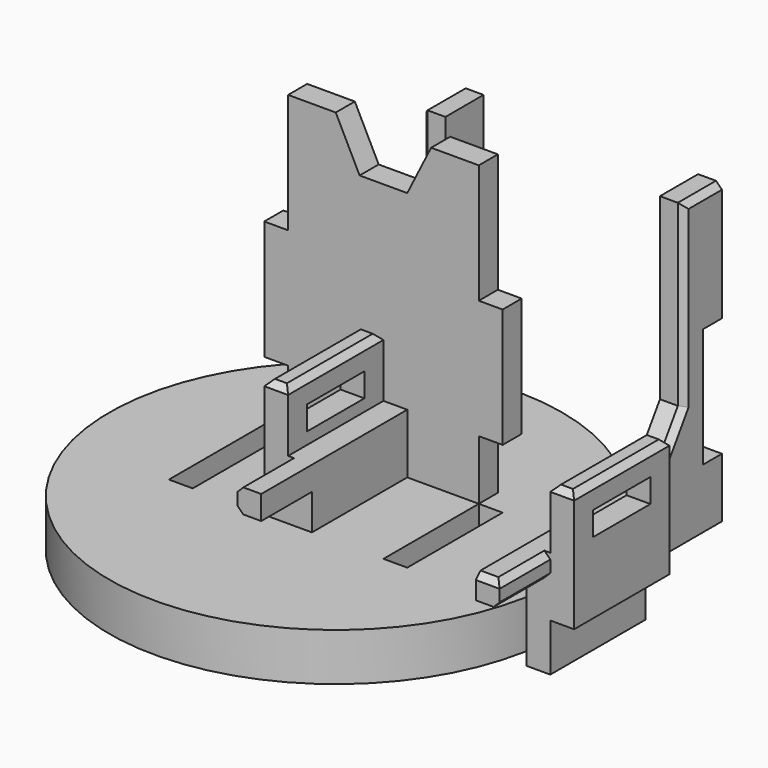
from build123d import *

# Parameters (mm, degrees)
F0_R       = 19
F1_DEPTH   = 4
F2_W       = 2
F2_H       = 10
F3_DEPTH   = 4.001
F5_DEPTH   = 2
F8_DEPTH   = 25
F9_W       = 2
F9_H       = 10
F9_H_2     = 5
F10_DEPTH  = 26.001
F6_W       = 2
F6_H       = 10
F11_DEPTH  = 19.001
F13_DEPTH  = 14.001
F15_W      = 10
F15_H      = 5
F16_DEPTH  = 2
F17_W      = 6
F17_H      = 2
F18_DEPTH  = 24.001
F19_W      = 10
F19_H      = 5
F20_DEPTH  = 2
F21_W      = 6
F21_H      = 2
F22_DEPTH  = 43.001
F23_SIZE   = 0.5
F23_2_SIZE = 0.5


with BuildPart() as f1:
    # F0 (on Top) → F1 (new body)
    with BuildSketch(Plane.XY):
        Circle(F0_R)
    extrude(amount=F1_DEPTH)

    # F2 (on face) → F3 (cut, through all)
    with BuildSketch(Plane.XY.offset(4)):
        with Locations((-9, 0)):
            Rectangle(F2_W, F2_H)
        with Locations((9, 0)):
            Rectangle(F2_W, F2_H)
    extrude(amount=-F3_DEPTH, mode=Mode.SUBTRACT)


with BuildPart() as f5:
    # F4 (on Right) → F5 (new body)
    with BuildSketch(Plane.YZ):
        Polygon((-5, 4), (-5, 0), (5, 0), (5, 4), (13, 4), (13, 29), (9, 29), (9, 14), (5.6833752096, 9), (-10.3166247904, 9), (-10.3166247904, 7), (-5, 7), align=None)
    extrude(amount=F5_DEPTH)

    # F6 (on face) → F11 (cut, through all)
    with BuildSketch(Plane(origin=(0, 0, 0), x_dir=(0, -1, 0), z_dir=(-1, 0, 0))):
        with Locations((-12, 14)):
            Rectangle(F6_W, F6_H)
    extrude(amount=-F11_DEPTH, mode=Mode.SUBTRACT)


with BuildPart() as f8:
    # F7 (on face) → F8 (new body)
    with BuildSketch(Plane.XY.offset(4)):
        Polygon((-10, 7), (-10, 5), (-8, 5), (8, 5), (10, 5), (10, 7), align=None)
    extrude(amount=F8_DEPTH)

    # F9 (on face) → F10 (cut, through all)
    with BuildSketch(Plane(origin=(0, 7, 0), x_dir=(-1, 0, 0), z_dir=(0, 1, 0))):
        with Locations((-9, 24)):
            Rectangle(F9_W, F9_H)
        with Locations((9, 24)):
            Rectangle(F9_W, F9_H)
        with Locations((9, 6.5)):
            Rectangle(F9_W, F9_H_2)
        with Locations((-9, 6.5)):
            Rectangle(F9_W, F9_H_2)
    extrude(amount=-F10_DEPTH, mode=Mode.SUBTRACT)

    # F12 (on face) → F13 (cut, through all)
    with BuildSketch(Plane.XZ.offset(-5)):
        Polygon((4, 29), (-4, 29), (-2, 25), (2, 25), align=None)
    extrude(amount=-F13_DEPTH, mode=Mode.SUBTRACT)


with BuildPart() as f14_1:
    # F14: copy of F5
    add(f5.part.moved(Location((20, 0, 0))))

    # F19 (on face) → F20 (join)
    with BuildSketch(Plane.YZ.offset(22)):
        with Locations((0, 11.5)):
            Rectangle(F19_W, F19_H)
        Polygon((-5, 4), (5, 4), (5, 9), (-5, 9), (-5, 7), align=None)
    extrude(amount=F20_DEPTH)

    # F21 (on face) → F22 (cut, through all)
    with BuildSketch(Plane.YZ.offset(24)):
        with Locations((0, 11)):
            Rectangle(F21_W, F21_H)
    extrude(amount=-F22_DEPTH, mode=Mode.SUBTRACT)

    # F23#2
    f23_2_edges = [f14_1.edges().sort_by_distance(p)[0] for p in [
        (24, 0, 14),
        (23, -5, 14),
        (23, 5, 14),
        (22, 0, 14),
        (22, -7.658312, 9),
        (21, -10.316625, 9),
        (22, 7.341688, 11.5),
        (22, 9, 21.5),
        (22, 11, 29),
        (22, -7.658312, 7),
    ]]
    chamfer(f23_2_edges, length=F23_2_SIZE)


with BuildPart() as f5_1:
    add(f5.part)

    # F15 (on face) → F16 (join)
    with BuildSketch(Plane(origin=(0, 0, 0), x_dir=(0, -1, 0), z_dir=(-1, 0, 0))):
        with Locations((0, 11.5)):
            Rectangle(F15_W, F15_H)
        Polygon((-5, 9), (-5, 4), (5, 4), (5, 7), (5, 9), align=None)
    extrude(amount=F16_DEPTH)

    # F17 (on face) → F18 (cut, through all)
    with BuildSketch(Plane(origin=(-2, 0, 0), x_dir=(0, -1, 0), z_dir=(-1, 0, 0))):
        with Locations((0, 11)):
            Rectangle(F17_W, F17_H)
    extrude(amount=-F18_DEPTH, mode=Mode.SUBTRACT)

    # F23
    f23_edges = [f5_1.edges().sort_by_distance(p)[0] for p in [
        (0, -7.658312, 9),
        (0, 0, 14),
        (-1, -5, 14),
        (-2, 0, 14),
        (-1, 5, 14),
        (0, 7.341688, 11.5),
        (0, 9, 21.5),
        (0, 11, 29),
        (0, -7.658312, 7),
    ]]
    chamfer(f23_edges, length=F23_SIZE)


solid = Compound([f1.part, f8.part, f14_1.part, f5_1.part])
